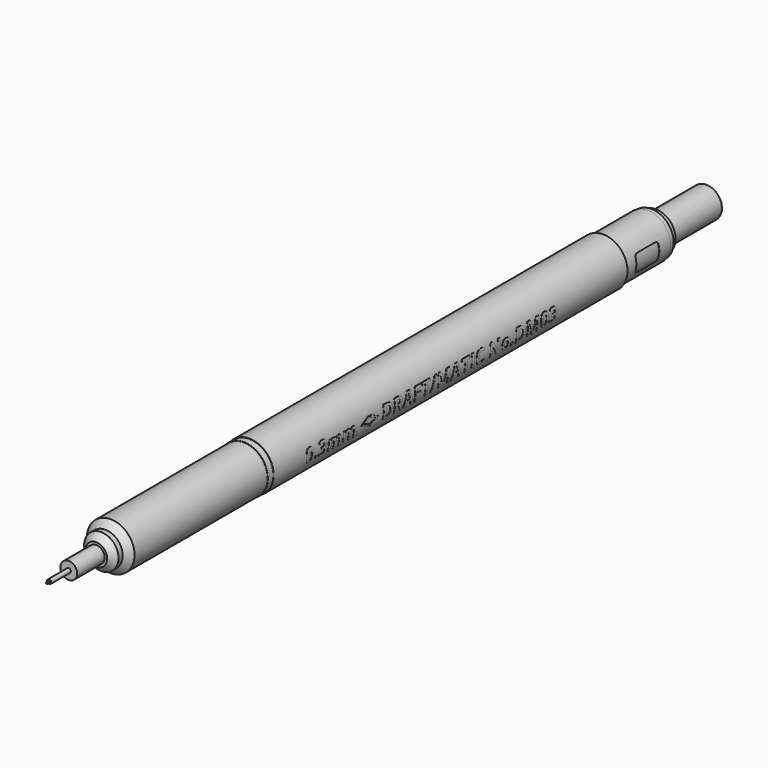
from build123d import *

# Parameters (mm, degrees)
F0_R          = 4.26
F1_DEPTH      = 77.1
F2_R          = 4.2
F3_DEPTH      = 1.2
F4_R          = 4.15
F5_DEPTH      = 29
F6_R          = 4.15
F7_DEPTH      = 1.15
F7_TAPER      = 45
F8_R          = 3
F9_DEPTH      = 0.9
F10_R         = 3
F11_DEPTH     = 1.1
F11_TAPER     = 45
F12_R         = 1.47
F13_DEPTH     = 6
F14_R         = 0.375
F15_DEPTH     = 4.25
F16_R         = 3.75
F17_DEPTH     = 9.5
F18_R         = 3.9
F19_DEPTH     = 1
F20_R         = 3.44
F21_DEPTH     = 1
F22_R         = 2.725
F23_DEPTH     = 11
F24_R         = 4
F24_R_2       = 3.95
F25_DEPTH     = 9.7
F28_DEPTH     = 1
F30_TEXT_SIZE = 3.2950779773
F31_DEPTH     = 1
F32_R         = 6
F32_R_2       = 4.3
F33_DEPTH     = 143.201
F34_R         = 0.15
F35_DEPTH     = 0.5


# Not quite as in the source:
# - Text() gives the source's letters only with a copy of the font that has no kerning and outlines rounded to 1/6400 em; it was checked with that copy


with BuildPart() as f1:
    # F0 (on Front) → F1 (new body)
    with BuildSketch(Plane.XZ):
        Circle(F0_R)
    extrude(amount=F1_DEPTH)


with BuildPart() as f3:
    # F2 (on face) → F3 (new body)
    with BuildSketch(Plane.XZ.offset(77.1)):
        Circle(F2_R)
    extrude(amount=F3_DEPTH)


with BuildPart() as f5:
    # F4 (on face) → F5 (new body)
    with BuildSketch(Plane.XZ.offset(78.3)):
        Circle(F4_R)
    extrude(amount=F5_DEPTH)


with BuildPart() as f7:
    # F6 (on face) → F7 (new body)
    with BuildSketch(Plane.XZ.offset(107.3)):
        Circle(F6_R)
    extrude(amount=F7_DEPTH, taper=F7_TAPER)

    # F8 (on face) → F9 (join)
    with BuildSketch(Plane.XZ.offset(108.45)):
        Circle(F8_R)
    extrude(amount=F9_DEPTH)

    # F10 (on face) → F11 (join)
    with BuildSketch(Plane.XZ.offset(109.35)):
        Circle(F10_R)
    extrude(amount=F11_DEPTH, taper=F11_TAPER)

    # F12 (on face) → F13 (join)
    with BuildSketch(Plane.XZ.offset(110.45)):
        Circle(F12_R)
    extrude(amount=F13_DEPTH)

    # F14 (on face) → F15 (join)
    with BuildSketch(Plane.XZ.offset(116.45)):
        Circle(F14_R)
    extrude(amount=F15_DEPTH)


with BuildPart() as f17:
    # F16 (on face) → F17 (new body)
    with BuildSketch(Plane(origin=(0, 0, 0), x_dir=(-1, 0, 0), z_dir=(0, 1, 0))):
        Circle(F16_R)
    extrude(amount=F17_DEPTH)


with BuildPart() as f19:
    # F18 (on face) → F19 (new body)
    with BuildSketch(Plane(origin=(0, 9.5, 0), x_dir=(-1, 0, 0), z_dir=(0, 1, 0))):
        Circle(F18_R)
    extrude(amount=F19_DEPTH)

    # F20 (on face) → F21 (join)
    with BuildSketch(Plane(origin=(0, 10.5, 0), x_dir=(-1, 0, 0), z_dir=(0, 1, 0))):
        Circle(F20_R)
    extrude(amount=F21_DEPTH)

    # F22 (on face) → F23 (join)
    with BuildSketch(Plane(origin=(0, 11.5, 0), x_dir=(-1, 0, 0), z_dir=(0, 1, 0))):
        Circle(F22_R)
    extrude(amount=F23_DEPTH)


with BuildPart() as f25:
    # F24 (on face) → F25 (new body)
    with BuildSketch(Plane(origin=(0, 0, 0), x_dir=(-1, 0, 0), z_dir=(0, 1, 0))):
        Circle(F24_R)
        Circle(F24_R_2, mode=Mode.SUBTRACT)
    extrude(amount=F25_DEPTH)

    # F27 (on offset) → F28 (cut)
    with BuildSketch(Plane.YZ.offset(4.2)):
        with BuildLine():
            ThreePointArc((7.25, 1), (7.1035533906, 1.3535533906), (6.75, 1.5))
            Line((6.75, 1.5), (2.75, 1.5))
            ThreePointArc((2.75, 1.5), (2.3964466094, 1.3535533906), (2.25, 1))
            Line((2.25, 1), (2.25, -1))
            ThreePointArc((2.25, -1), (2.3964466094, -1.3535533906), (2.75, -1.5))
            Line((2.75, -1.5), (6.75, -1.5))
            ThreePointArc((6.75, -1.5), (7.1035533906, -1.3535533906), (7.25, -1))
            Line((7.25, -1), (7.25, 1))
        make_face()
    extrude(amount=-F28_DEPTH, mode=Mode.SUBTRACT)


with BuildPart() as f31:
    # F30 (on offset) → F31 (new body)
    with BuildSketch(Plane.YZ.offset(5)):
        with Locations((-70.1, -1.3288366687)):
            Text('0.3mm <> DRAFT/MATIC No.DM03', F30_TEXT_SIZE, font='Open Sans', font_style=FontStyle.BOLD, text_align=(TextAlign.LEFT, TextAlign.BOTTOM))
    extrude(amount=-F31_DEPTH)

    # F32 (on face) → F33 (cut, through all)
    with BuildSketch(Plane(origin=(0, 22.5, 0), x_dir=(-1, 0, 0), z_dir=(0, 1, 0))):
        Circle(F32_R)
        Circle(F32_R_2, mode=Mode.SUBTRACT)
    extrude(amount=-F33_DEPTH, mode=Mode.SUBTRACT)


with BuildPart() as f35:
    # F34 (on face) → F35 (new body)
    with BuildSketch(Plane.XZ.offset(120.7)):
        Circle(F34_R)
    extrude(amount=F35_DEPTH)


solid = Compound([f1.part, f3.part, f5.part, f7.part, f17.part, f19.part, f25.part, f31.part, f35.part])
